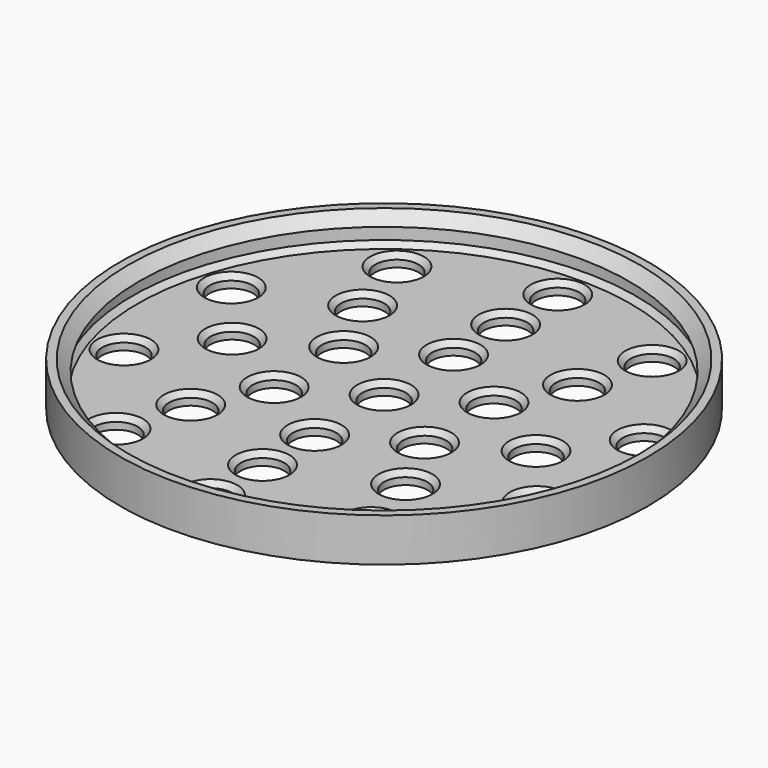
from build123d import *

# Parameters (mm, degrees)
F0_R     = 19.304
F0_R_2   = 1.5875
F1_DEPTH = 3.175
F2_T     = -0.889
F3_DEPTH = 3.176
F4_R     = 18.415
F4_R_2   = 17.907
F5_DEPTH = 0.79375
F6_SIZE  = 0.79374
F7_SIZE  = 0.381


# Not quite as in the source:
# - a fillet or chamfer is up to 0.001 mm smaller than in the source, because OpenCascade refuses the exact size
# - a feature names something its author has since deleted; it is built from what else it names


with BuildPart() as f1:
    # F0 (on Top) → F1 (new body)
    with BuildSketch(Plane.XY):
        Circle(F0_R)
        with Locations((-9.3310908801, -12.8431447857)):
            Circle(F0_R_2, mode=Mode.SUBTRACT)
        with Locations((-15.0980221962, -4.9056447857)):
            Circle(F0_R_2, mode=Mode.SUBTRACT)
        with Locations((-7.8577241059, -7.8577241059)):
            Circle(F0_R_2, mode=Mode.SUBTRACT)
        with Locations((-5.499261314, -3.175)):
            Circle(F0_R_2, mode=Mode.SUBTRACT)
        with Locations((0, -15.875)):
            Circle(F0_R_2, mode=Mode.SUBTRACT)
        with Locations((0, -11.1125)):
            Circle(F0_R_2, mode=Mode.SUBTRACT)
        with Locations((9.3310908801, -12.8431447857)):
            Circle(F0_R_2, mode=Mode.SUBTRACT)
        with Locations((0, -6.35)):
            Circle(F0_R_2, mode=Mode.SUBTRACT)
        with Locations((7.8577241059, -7.8577241059)):
            Circle(F0_R_2, mode=Mode.SUBTRACT)
        with Locations((5.499261314, -3.175)):
            Circle(F0_R_2, mode=Mode.SUBTRACT)
        with Locations((15.0980221962, -4.9056447857)):
            Circle(F0_R_2, mode=Mode.SUBTRACT)
        with Locations((-11.1125, 0)):
            Circle(F0_R_2, mode=Mode.SUBTRACT)
        with Locations((-15.0980221962, 4.9056447857)):
            Circle(F0_R_2, mode=Mode.SUBTRACT)
        with Locations((-5.499261314, 3.175)):
            Circle(F0_R_2, mode=Mode.SUBTRACT)
        with Locations((-7.8577241059, 7.8577241059)):
            Circle(F0_R_2, mode=Mode.SUBTRACT)
        with Locations((-9.3310908801, 12.8431447857)):
            Circle(F0_R_2, mode=Mode.SUBTRACT)
        Circle(F0_R_2, mode=Mode.SUBTRACT)
        with Locations((5.499261314, 3.175)):
            Circle(F0_R_2, mode=Mode.SUBTRACT)
        with Locations((0, 6.35)):
            Circle(F0_R_2, mode=Mode.SUBTRACT)
        with Locations((7.8577241059, 7.8577241059)):
            Circle(F0_R_2, mode=Mode.SUBTRACT)
        with Locations((11.1125, 0)):
            Circle(F0_R_2, mode=Mode.SUBTRACT)
        with Locations((15.0980221962, 4.9056447857)):
            Circle(F0_R_2, mode=Mode.SUBTRACT)
        with Locations((0, 11.1125)):
            Circle(F0_R_2, mode=Mode.SUBTRACT)
        with Locations((9.3310908801, 12.8431447857)):
            Circle(F0_R_2, mode=Mode.SUBTRACT)
        with Locations((0, 15.875)):
            Circle(F0_R_2, mode=Mode.SUBTRACT)
        Circle(F0_R_2)
        with Locations((5.499261314, 3.175)):
            Circle(F0_R_2)
        with Locations((0, 15.875)):
            Circle(F0_R_2)
        with Locations((0, 11.1125)):
            Circle(F0_R_2)
        with Locations((0, 6.35)):
            Circle(F0_R_2)
        with Locations((-9.3310908801, 12.8431447857)):
            Circle(F0_R_2)
        with Locations((-7.8577241059, 7.8577241059)):
            Circle(F0_R_2)
        with Locations((-15.0980221962, 4.9056447857)):
            Circle(F0_R_2)
        with Locations((-11.1125, 0)):
            Circle(F0_R_2)
        with Locations((-5.499261314, 3.175)):
            Circle(F0_R_2)
        with Locations((-15.0980221962, -4.9056447857)):
            Circle(F0_R_2)
        with Locations((-7.8577241059, -7.8577241059)):
            Circle(F0_R_2)
        with Locations((-5.499261314, -3.175)):
            Circle(F0_R_2)
        with Locations((-9.3310908801, -12.8431447857)):
            Circle(F0_R_2)
        with Locations((0, -11.1125)):
            Circle(F0_R_2)
        with Locations((0, -15.875)):
            Circle(F0_R_2)
        with Locations((0, -6.35)):
            Circle(F0_R_2)
        with Locations((7.8577241059, -7.8577241059)):
            Circle(F0_R_2)
        with Locations((9.3310908801, -12.8431447857)):
            Circle(F0_R_2)
        with Locations((15.0980221962, -4.9056447857)):
            Circle(F0_R_2)
        with Locations((11.1125, 0)):
            Circle(F0_R_2)
        with Locations((5.499261314, -3.175)):
            Circle(F0_R_2)
        with Locations((7.8577241059, 7.8577241059)):
            Circle(F0_R_2)
        with Locations((15.0980221962, 4.9056447857)):
            Circle(F0_R_2)
        with Locations((9.3310908801, 12.8431447857)):
            Circle(F0_R_2)
    extrude(amount=F1_DEPTH)

    # F2
    f2_openings = [f1.faces().sort_by_distance(p)[0] for p in [
        (0, 0, 3.175),
    ]]
    offset(amount=F2_T, openings=f2_openings)

    # F0 (on Top) → F3 (cut, through all)
    with BuildSketch(Plane.XY):
        with Locations((0, -6.35)):
            Circle(F0_R_2)
        with Locations((7.8577241059, -7.8577241059)):
            Circle(F0_R_2)
        with Locations((9.3310908801, -12.8431447857)):
            Circle(F0_R_2)
        with Locations((0, -11.1125)):
            Circle(F0_R_2)
        with Locations((0, -15.875)):
            Circle(F0_R_2)
        with Locations((-9.3310908801, -12.8431447857)):
            Circle(F0_R_2)
        with Locations((-7.8577241059, -7.8577241059)):
            Circle(F0_R_2)
        with Locations((-5.499261314, -3.175)):
            Circle(F0_R_2)
        with Locations((-15.0980221962, -4.9056447857)):
            Circle(F0_R_2)
        with Locations((-11.1125, 0)):
            Circle(F0_R_2)
        with Locations((-5.499261314, 3.175)):
            Circle(F0_R_2)
        with Locations((-15.0980221962, 4.9056447857)):
            Circle(F0_R_2)
        with Locations((-9.3310908801, 12.8431447857)):
            Circle(F0_R_2)
        with Locations((-7.8577241059, 7.8577241059)):
            Circle(F0_R_2)
        with Locations((0, 15.875)):
            Circle(F0_R_2)
        with Locations((0, 11.1125)):
            Circle(F0_R_2)
        with Locations((0, 6.35)):
            Circle(F0_R_2)
        with Locations((5.499261314, 3.175)):
            Circle(F0_R_2)
        with Locations((9.3310908801, 12.8431447857)):
            Circle(F0_R_2)
        with Locations((7.8577241059, 7.8577241059)):
            Circle(F0_R_2)
        with Locations((5.499261314, -3.175)):
            Circle(F0_R_2)
        with Locations((15.0980221962, 4.9056447857)):
            Circle(F0_R_2)
        with Locations((15.0980221962, -4.9056447857)):
            Circle(F0_R_2)
        with Locations((11.1125, 0)):
            Circle(F0_R_2)
        Circle(F0_R_2)
    extrude(amount=F3_DEPTH, mode=Mode.SUBTRACT)

    # F4 (on face) → F5 (join)
    with BuildSketch(Plane.XY.offset(3.175)):
        Circle(F4_R)
        Circle(F4_R_2, mode=Mode.SUBTRACT)
    extrude(amount=-F5_DEPTH)

    # F6 (size 0.79375 in the source; OpenCascade refuses exactly that, so slightly less here)
    f6_edges = [f1.edges().sort_by_distance(p)[0] for p in [
        (-17.907, 0, 3.175),
    ]]
    chamfer(f6_edges, length=F6_SIZE)

    # F7
    f7_edges = [f1.edges().sort_by_distance(p)[0] for p in [
        (-18.415, 0, 0.889),
        (18.415, 0, 1.635125),
        (-10.918591, -12.843145, 0.889),
        (-16.685522, -4.905645, 0.889),
        (-9.445224, -7.857724, 0.889),
        (-7.086761, -3.175, 0.889),
        (-1.5875, -15.875, 0.889),
        (-1.5875, -11.1125, 0.889),
        (7.743591, -12.843145, 0.889),
        (-1.5875, -6.35, 0.889),
        (6.270224, -7.857724, 0.889),
        (3.911761, -3.175, 0.889),
        (13.510522, -4.905645, 0.889),
        (-12.7, 0, 0.889),
        (-16.685522, 4.905645, 0.889),
        (-7.086761, 3.175, 0.889),
        (-9.445224, 7.857724, 0.889),
        (-10.918591, 12.843145, 0.889),
        (-1.5875, 0, 0.889),
        (3.911761, 3.175, 0.889),
        (-1.5875, 6.35, 0.889),
        (6.270224, 7.857724, 0.889),
        (9.525, 0, 0.889),
        (13.510522, 4.905645, 0.889),
        (-1.5875, 11.1125, 0.889),
        (-1.5875, 15.875, 0.889),
        (7.743591, 12.843145, 0.889),
    ]]
    chamfer(f7_edges, length=F7_SIZE)


solid = f1.part
